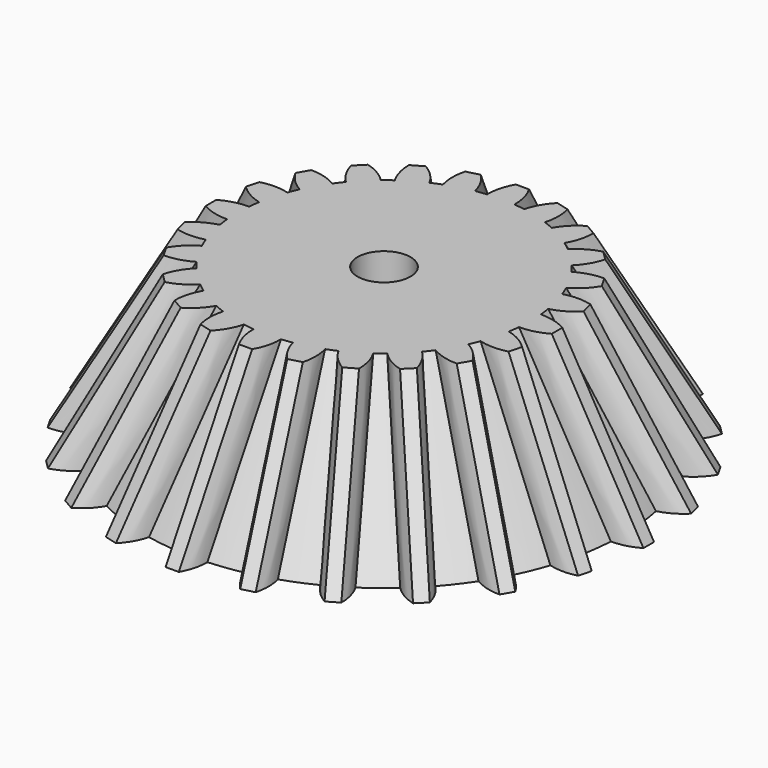
from build123d import *

# Parameters (mm, degrees)
F4_COPIES_COUNT = 24


# Not quite as in the source:
# - a pattern or mirror of a feature is missing from the dataset's text; its kind, count and spacing are read off the source's solid


with BuildPart() as f1:
    # F0 (on Front) → F1 (revolve)
    with BuildSketch(Plane.XZ):
        Polygon((35.1529547439, 38.1), (6.35, 38.1), (6.35, 0), (57.15, 0), align=None)
    revolve(axis=Axis((0, 0, 34.2554152012), (0, 0, 1)))

    # F4: sweep along a path in F3
    with BuildLine(Plane.YZ) as f4_path:
        Line((-57.15, 0), (-35.1529547439, 38.1))
    # F2 (on face) → F4 (sweep)
    with BuildSketch(Plane.XY.offset(38.1)):
        with BuildLine():
            Line((-1.5875, -41.5029547439), (0, -41.5029547439))
            Line((0, -41.5029547439), (0, -35.1529547439))
            ThreePointArc((0, -35.1529547439), (-1.6458259699, -35.1144056493), (-3.2880422802, -34.9988429121))
            ThreePointArc((-3.2880422802, -34.9988429121), (-2.8759534621, -38.3654644419), (-1.5875, -41.5029547439))
        make_face()
        with BuildLine():
            Line((0, -35.1529547439), (0, -41.5029547439))
            Line((0, -41.5029547439), (1.5875, -41.5029547439))
            ThreePointArc((1.5875, -41.5029547439), (2.8759534621, -38.3654644419), (3.2880422802, -34.9988429121))
            ThreePointArc((3.2880422802, -34.9988429121), (1.6458259699, -35.1144056493), (0, -35.1529547439))
        make_face()
    f4 = sweep(path=f4_path.line)

    # F4_copies: F4 ×24 about axis
    f4_copies_axis = Axis((0, 0, 0), (0, 0, 1))
    for i in range(1, F4_COPIES_COUNT):
        add(f4.rotate(f4_copies_axis, i * 360 / F4_COPIES_COUNT))


solid = f1.part
